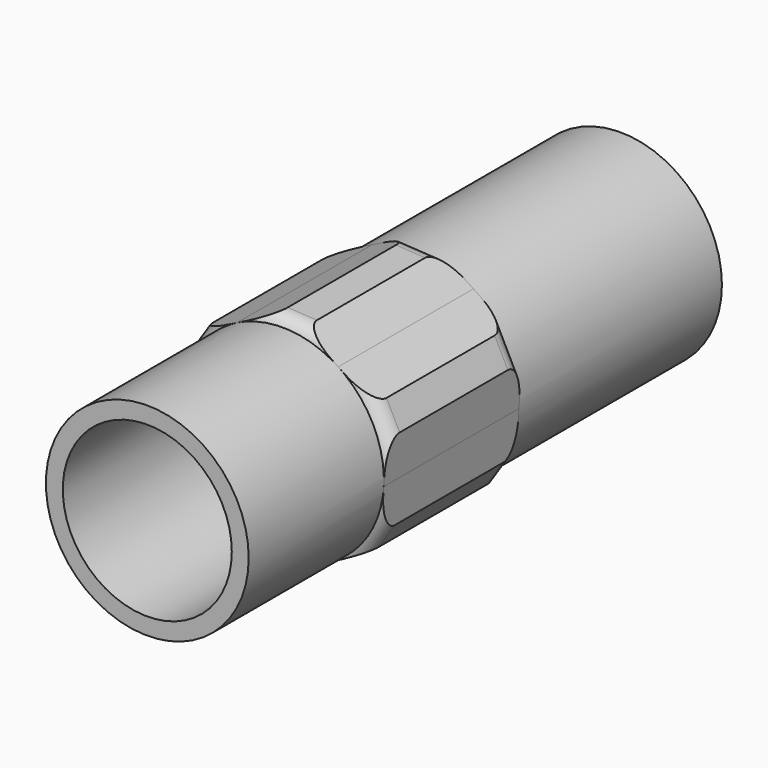
from build123d import *

# Parameters (mm, degrees)
F0_R         = 7.62
F1_DEPTH     = 19.05
F3_DEPTH     = 12.7
F4_SIZE      = 1.27
F5_T1_DEPTH  = 8.5497045256
F5_T3_DEPTH  = 8.5497045256
F5_T5_DEPTH  = 8.5497045256
F5_T7_DEPTH  = 8.5497045256
F5_T12_DEPTH = 8.5497045256
F5_S13_R     = 7.62
F5_T14_DEPTH = 6
F5_T18_DEPTH = 8.5497045256
F5_S19_R     = 7.62
F5_T20_DEPTH = 6
F5_T24_DEPTH = 8.5497045256
F5_S25_R     = 7.62
F5_T26_DEPTH = 6
F5_T30_DEPTH = 8.5497045256
F5_S31_R     = 7.62
F5_T32_DEPTH = 6
F5_T36_DEPTH = 8.5497045256
F5_S37_R     = 7.62
F5_T38_DEPTH = 6
F5_T42_DEPTH = 8.5497045256
F5_S43_R     = 7.62
F5_T44_DEPTH = 6
F6_R         = 7.62
F7_DEPTH     = 12.7
F8_R         = 6.35
F9_DEPTH     = 44.4510001


# Not quite as in the source:
# - a fillet or chamfer that OpenCascade refuses, or shapes differently, is made with other operations: its cross-section is extruded or revolved along the edge and cut away or added


with BuildPart() as f1:
    # F0 (on Front) → F1 (new body)
    with BuildSketch(Plane.XZ):
        Circle(F0_R)
    extrude(amount=F1_DEPTH)

    # F2 (on face) → F3 (join)
    with BuildSketch(Plane.XZ.offset(19.05)):
        with BuildLine():
            Line((7.8629215405, 3.9488814679), (4.1872753391, 6.3664059904))
            ThreePointArc((4.1872753391, 6.3664059904), (6.7071394083, 3.6164459015), (7.62, 0))
            ThreePointArc((7.62, 0), (7.616776064, -0.2216357159), (7.6071069841, -0.4430838887))
            Line((7.6071069841, -0.4430838887), (7.8629215405, 3.9488814679))
        make_face()
        with BuildLine():
            ThreePointArc((4.1872753391, 6.3664059904), (0.4430838236, 7.6071069879), (-3.4198316443, 6.8094898138))
            ThreePointArc((-3.4198316443, 6.8094898138), (-6.3664059346, 4.187275424), (-7.6071069765, 0.4430840189))
            ThreePointArc((-7.6071069765, 0.4430840189), (-6.8094898664, -3.4198315396), (-4.187275378, -6.3664059648))
            ThreePointArc((-4.187275378, -6.3664059648), (-0.4430838337, -7.6071069873), (3.419831668, -6.8094898019))
            ThreePointArc((3.419831668, -6.8094898019), (6.3664059777, -4.1872753585), (7.6071069841, -0.4430838887))
            ThreePointArc((7.6071069841, -0.4430838887), (7.616776064, -0.2216357159), (7.62, 0))
            ThreePointArc((7.62, 0), (6.7071394083, 3.6164459015), (4.1872753391, 6.3664059904))
        make_face()
        with BuildLine():
            ThreePointArc((7.6071069841, -0.4430838887), (6.3664059777, -4.1872753585), (3.419831668, -6.8094898019))
            Line((3.419831668, -6.8094898019), (7.351292438, -4.8350490681))
            Line((7.351292438, -4.8350490681), (7.6071069841, -0.4430838887))
        make_face()
        with BuildLine():
            ThreePointArc((3.419831668, -6.8094898019), (-0.4430838337, -7.6071069873), (-4.187275378, -6.3664059648))
            Line((-4.187275378, -6.3664059648), (-0.5116291025, -8.783930536))
            Line((-0.5116291025, -8.783930536), (3.419831668, -6.8094898019))
        make_face()
        with BuildLine():
            ThreePointArc((-4.187275378, -6.3664059648), (-6.8094898664, -3.4198315396), (-7.6071069765, 0.4430840189))
            Line((-7.6071069765, 0.4430840189), (-7.8629215405, -3.9488814679))
            Line((-7.8629215405, -3.9488814679), (-4.187275378, -6.3664059648))
        make_face()
        with BuildLine():
            Line((-3.4198316443, 6.8094898138), (-7.351292438, 4.8350490681))
            Line((-7.351292438, 4.8350490681), (-7.6071069765, 0.4430840189))
            ThreePointArc((-7.6071069765, 0.4430840189), (-6.3664059346, 4.187275424), (-3.4198316443, 6.8094898138))
        make_face()
        with BuildLine():
            Line((0.5116291025, 8.783930536), (-3.4198316443, 6.8094898138))
            ThreePointArc((-3.4198316443, 6.8094898138), (0.4430838236, 7.6071069879), (4.1872753391, 6.3664059904))
            Line((4.1872753391, 6.3664059904), (0.5116291025, 8.783930536))
        make_face()
    extrude(amount=F3_DEPTH)

    # F4
    f4_edges = [f1.edges().sort_by_distance(p)[0] for p in [
        (7.862922, -25.4, 3.948881),
        (7.351292, -25.4, -4.835049),
        (-0.511629, -25.4, -8.783931),
        (-7.862922, -25.4, -3.948881),
        (-7.351292, -25.4, 4.835049),
        (0.511629, -25.4, 8.783931),
    ]]
    chamfer(f4_edges, length=F4_SIZE)

    # F5: fillet of radius 1.27 on 12 edges, made by hand

    # F5_s2 → F5_t1 (cut)
    with BuildSketch(Plane(origin=(1.918540045, 0, -3.8201526101), x_dir=(0, 1, 0), z_dir=(-0.4487968068, 0, 0.8936338323))):
        with BuildLine():
            ThreePointArc((-30.48, -8.1638181024), (-31.3780256121, -7.7918437146), (-31.75, -6.8938181024))
            Line((-31.75, -6.8938181024), (-31.75, -8.1638181024))
            Line((-31.75, -8.1638181024), (-30.48, -8.1638181024))
        make_face()
        with BuildLine():
            ThreePointArc((-31.75, 6.8938181024), (-31.3780256121, 7.7918437146), (-30.48, 8.1638181024))
            Line((-30.48, 8.1638181024), (-31.75, 8.1638181024))
            Line((-31.75, 8.1638181024), (-31.75, 6.8938181024))
        make_face()
    extrude(amount=F5_T1_DEPTH, mode=Mode.SUBTRACT)

    # F5_s4 → F5_t3 (cut)
    with BuildSketch(Plane(origin=(4.2676192292, 0, -0.2485718879), x_dir=(0, 1, 0), z_dir=(-0.9983080038, 0, 0.0581474803))):
        with BuildLine():
            ThreePointArc((-31.75, -6.8938181024), (-31.3780256121, -7.7918437146), (-30.48, -8.1638181024))
            Line((-30.48, -8.1638181024), (-31.75, -8.1638181024))
            Line((-31.75, -8.1638181024), (-31.75, -6.8938181024))
        make_face()
        with BuildLine():
            ThreePointArc((-31.75, 6.8938181024), (-31.3780256121, 7.7918437146), (-30.48, 8.1638181024))
            Line((-30.48, 8.1638181024), (-31.75, 8.1638181024))
            Line((-31.75, 8.1638181024), (-31.75, 6.8938181024))
        make_face()
    extrude(amount=F5_T3_DEPTH, mode=Mode.SUBTRACT)

    # F5_s6 → F5_t5 (cut)
    with BuildSketch(Plane(origin=(-2.3490791841, 0, -3.5715807222), x_dir=(0, 1, 0), z_dir=(0.5495111971, 0, 0.835486352))):
        with BuildLine():
            ThreePointArc((-31.75, 6.8938181024), (-31.3780256121, 7.7918437146), (-30.48, 8.1638181024))
            Line((-30.48, 8.1638181024), (-31.75, 8.1638181024))
            Line((-31.75, 8.1638181024), (-31.75, 6.8938181024))
        make_face()
    extrude(amount=F5_T5_DEPTH, mode=Mode.SUBTRACT)

    # F5_s8 → F5_t7 (cut)
    with BuildSketch(Plane(origin=(2.3490791841, 0, 3.5715807222), x_dir=(0, 1, 0), z_dir=(-0.5495111971, 0, -0.835486352))):
        with BuildLine():
            ThreePointArc((-30.48, 8.1638181024), (-31.3780256121, 7.7918437146), (-31.75, 6.8938181024))
            Line((-31.75, 6.8938181024), (-31.75, 8.1638181024))
            Line((-31.75, 8.1638181024), (-30.48, 8.1638181024))
        make_face()
    extrude(amount=F5_T7_DEPTH, mode=Mode.SUBTRACT)


with BuildPart() as f5_tool10:
    # F5_s11 → F5_t12 (new body)
    with BuildSketch(Plane(origin=(4.2676192292, 0, -0.2485718879), x_dir=(0, 1, 0), z_dir=(-0.9983080038, 0, 0.0581474803))):
        with BuildLine():
            ThreePointArc((-19.05, -6.8938181024), (-19.4219743879, -7.7918437146), (-20.32, -8.1638181024))
            Line((-20.32, -8.1638181024), (-19.05, -8.1638181024))
            Line((-19.05, -8.1638181024), (-19.05, -6.8938181024))
        make_face()
    extrude(amount=F5_T12_DEPTH)

    # F5_s13 → F5_t14 (cut, symmetric)
    with BuildSketch(Plane.XZ.offset(19.7)):
        Circle(F5_S13_R)
    extrude(amount=F5_T14_DEPTH, both=True, mode=Mode.SUBTRACT)


with BuildPart() as f1_1:
    add(f1.part)

    # F5_t9: cut F5_tool10
    add(f5_tool10.part, mode=Mode.SUBTRACT)


with BuildPart() as f5_tool16:
    # F5_s17 → F5_t18 (new body)
    with BuildSketch(Plane(origin=(-2.3490791841, 0, -3.5715807222), x_dir=(0, 1, 0), z_dir=(0.5495111971, 0, 0.835486352))):
        with BuildLine():
            ThreePointArc((-19.05, 6.8938181024), (-19.4219743879, 7.7918437146), (-20.32, 8.1638181024))
            Line((-20.32, 8.1638181024), (-19.05, 8.1638181024))
            Line((-19.05, 8.1638181024), (-19.05, 6.8938181024))
        make_face()
    extrude(amount=F5_T18_DEPTH)

    # F5_s19 → F5_t20 (cut, symmetric)
    with BuildSketch(Plane.XZ.offset(19.7)):
        Circle(F5_S19_R)
    extrude(amount=F5_T20_DEPTH, both=True, mode=Mode.SUBTRACT)


with BuildPart() as f1_2:
    add(f1_1.part)

    # F5_t15: cut F5_tool16
    add(f5_tool16.part, mode=Mode.SUBTRACT)


with BuildPart() as f5_tool22:
    # F5_s23 → F5_t24 (new body)
    with BuildSketch(Plane(origin=(1.918540045, 0, -3.8201526101), x_dir=(0, 1, 0), z_dir=(-0.4487968068, 0, 0.8936338323))):
        with BuildLine():
            ThreePointArc((-19.05, 6.8938181024), (-19.4219743879, 7.7918437146), (-20.32, 8.1638181024))
            Line((-20.32, 8.1638181024), (-19.05, 8.1638181024))
            Line((-19.05, 8.1638181024), (-19.05, 6.8938181024))
        make_face()
    extrude(amount=F5_T24_DEPTH)

    # F5_s25 → F5_t26 (cut, symmetric)
    with BuildSketch(Plane.XZ.offset(19.7)):
        Circle(F5_S25_R)
    extrude(amount=F5_T26_DEPTH, both=True, mode=Mode.SUBTRACT)


with BuildPart() as f1_3:
    add(f1_2.part)

    # F5_t21: cut F5_tool22
    add(f5_tool22.part, mode=Mode.SUBTRACT)


with BuildPart() as f5_tool28:
    # F5_s29 → F5_t30 (new body)
    with BuildSketch(Plane(origin=(4.2676192292, 0, -0.2485718879), x_dir=(0, 1, 0), z_dir=(-0.9983080038, 0, 0.0581474803))):
        with BuildLine():
            ThreePointArc((-19.05, 6.8938181024), (-19.4219743879, 7.7918437146), (-20.32, 8.1638181024))
            Line((-20.32, 8.1638181024), (-19.05, 8.1638181024))
            Line((-19.05, 8.1638181024), (-19.05, 6.8938181024))
        make_face()
    extrude(amount=F5_T30_DEPTH)

    # F5_s31 → F5_t32 (cut, symmetric)
    with BuildSketch(Plane.XZ.offset(19.7)):
        Circle(F5_S31_R)
    extrude(amount=F5_T32_DEPTH, both=True, mode=Mode.SUBTRACT)


with BuildPart() as f1_4:
    add(f1_3.part)

    # F5_t27: cut F5_tool28
    add(f5_tool28.part, mode=Mode.SUBTRACT)


with BuildPart() as f5_tool34:
    # F5_s35 → F5_t36 (new body)
    with BuildSketch(Plane(origin=(2.3490791841, 0, 3.5715807222), x_dir=(0, 1, 0), z_dir=(-0.5495111971, 0, -0.835486352))):
        with BuildLine():
            ThreePointArc((-19.05, 6.8938181024), (-19.4219743879, 7.7918437146), (-20.32, 8.1638181024))
            Line((-20.32, 8.1638181024), (-19.05, 8.1638181024))
            Line((-19.05, 8.1638181024), (-19.05, 6.8938181024))
        make_face()
    extrude(amount=F5_T36_DEPTH)

    # F5_s37 → F5_t38 (cut, symmetric)
    with BuildSketch(Plane.XZ.offset(19.7)):
        Circle(F5_S37_R)
    extrude(amount=F5_T38_DEPTH, both=True, mode=Mode.SUBTRACT)


with BuildPart() as f1_5:
    add(f1_4.part)

    # F5_t33: cut F5_tool34
    add(f5_tool34.part, mode=Mode.SUBTRACT)


with BuildPart() as f5_tool40:
    # F5_s41 → F5_t42 (new body)
    with BuildSketch(Plane(origin=(1.918540045, 0, -3.8201526101), x_dir=(0, 1, 0), z_dir=(-0.4487968068, 0, 0.8936338323))):
        with BuildLine():
            ThreePointArc((-19.05, -6.8938181024), (-19.4219743879, -7.7918437146), (-20.32, -8.1638181024))
            Line((-20.32, -8.1638181024), (-19.05, -8.1638181024))
            Line((-19.05, -8.1638181024), (-19.05, -6.8938181024))
        make_face()
    extrude(amount=F5_T42_DEPTH)

    # F5_s43 → F5_t44 (cut, symmetric)
    with BuildSketch(Plane.XZ.offset(19.7)):
        Circle(F5_S43_R)
    extrude(amount=F5_T44_DEPTH, both=True, mode=Mode.SUBTRACT)


with BuildPart() as f1_6:
    add(f1_5.part)

    # F5_t39: cut F5_tool40
    add(f5_tool40.part, mode=Mode.SUBTRACT)

    # F6 (on face) → F7 (join)
    with BuildSketch(Plane.XZ.offset(31.75)):
        Circle(F6_R)
    extrude(amount=F7_DEPTH)

    # F8 (on face) → F9 (cut, through all)
    with BuildSketch(Plane.XZ.offset(44.45)):
        Circle(F8_R)
    extrude(amount=-F9_DEPTH, mode=Mode.SUBTRACT)


solid = f1_6.part
